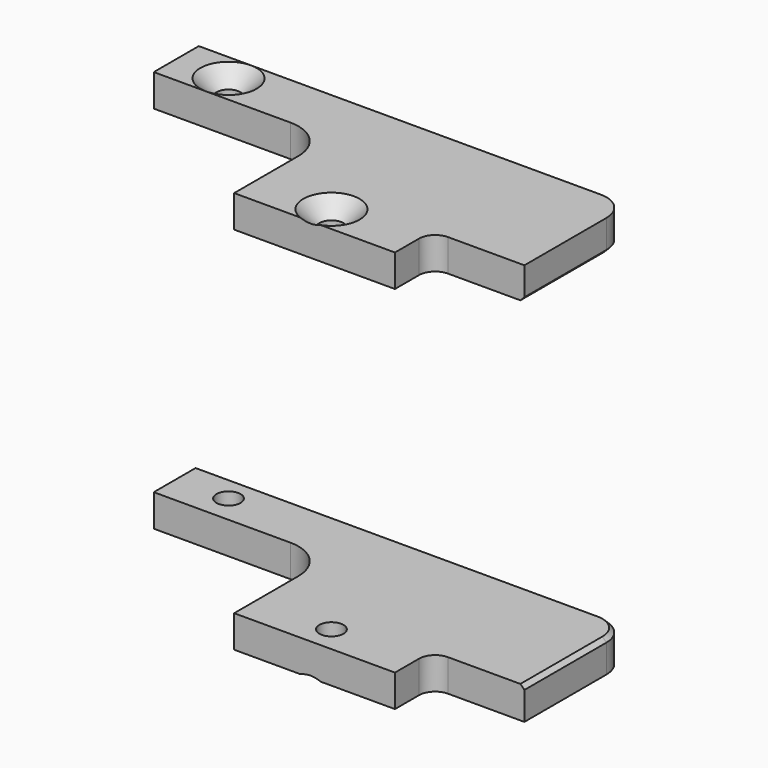
from build123d import *

# Parameters (mm, degrees)
F0_W      = 42
F0_H      = 22
F1_DEPTH  = 4
F2_W      = 29
F2_H      = 16.25
F3_DEPTH  = 4
F4_R      = 3.5
F5_R      = 2
F6_R      = 1.5
F7_DEPTH  = 25
F8_W      = 22
F8_H      = 15
F9_DEPTH  = 25
F10_R     = 5
F11_R     = 1.5
F12_DEPTH = 25
F15_SIZE  = 0.5


# Not quite as in the source:
# - a fillet or chamfer that OpenCascade refuses, or shapes differently, is made with other operations: its cross-section is extruded or revolved along the edge and cut away or added


with BuildPart() as f1:
    # F0 (on Top) → F1 (new body)
    with BuildSketch(Plane.XY):
        with Locations((21, -11)):
            Rectangle(F0_W, F0_H)
    extrude(amount=F1_DEPTH)

    # F2 (on Top) → F3 (join)
    with BuildSketch(Plane.XY):
        with Locations((39, -8.125)):
            Rectangle(F2_W, F2_H)
    extrude(amount=F3_DEPTH)

    # F4
    f4_edges = [f1.edges().sort_by_distance(p)[0] for p in [
        (53.5, 0, 2),
    ]]
    fillet(f4_edges, radius=F4_R)

    # F5
    f5_edges = [f1.edges().sort_by_distance(p)[0] for p in [
        (42, -16.25, 2),
    ]]
    fillet(f5_edges, radius=F5_R)

    # F6 (on face) → F7 (cut)
    with BuildSketch(Plane.XY.offset(4)):
        with Locations((6.5, -3.5)):
            Circle(F6_R)
    extrude(amount=-F7_DEPTH, mode=Mode.SUBTRACT)

    # F8 (on face) → F9 (cut)
    with BuildSketch(Plane.XY.offset(4)):
        with Locations((11, -14.5)):
            Rectangle(F8_W, F8_H)
    extrude(amount=-F9_DEPTH, mode=Mode.SUBTRACT)

    # F10
    f10_edges = [f1.edges().sort_by_distance(p)[0] for p in [
        (22, -7, 2),
    ]]
    fillet(f10_edges, radius=F10_R)

    # F11 (on face) → F12 (cut)
    with BuildSketch(Plane.XY.offset(4)):
        with Locations((31.5, -18.75)):
            Circle(F11_R)
    extrude(amount=-F12_DEPTH, mode=Mode.SUBTRACT)

    # F14: chamfer of 2 on 2 edges, made by hand

    # F14_s1 → F14_t2 (revolve, cut)
    with BuildSketch(Plane.XZ.offset(18.75)):
        Polygon((35, 0), (33, 2), (33, 0), align=None)
    revolve(axis=Axis((31.5, -18.75, 0), (0, 0, 1)), mode=Mode.SUBTRACT)

    # F14_s3 → F14_t4 (revolve, cut)
    with BuildSketch(Plane.XZ.offset(3.5)):
        Polygon((10, 0), (8, 2), (8, 0), align=None)
    revolve(axis=Axis((6.5, -3.5, 0), (0, 0, 1)), mode=Mode.SUBTRACT)

    # F15
    f15_edges = [f1.edges().sort_by_distance(p)[0] for p in [
        (53.5, -9.875, 4),
        (52.474874, -1.025126, 4),
        (25, 0, 4),
    ]]
    chamfer(f15_edges, length=F15_SIZE)


with BuildPart() as f16_1:
    # F16: instance of F1
    add(f1.part.mirror(Plane.XY.offset(25)))


solid = Compound([f1.part, f16_1.part])
